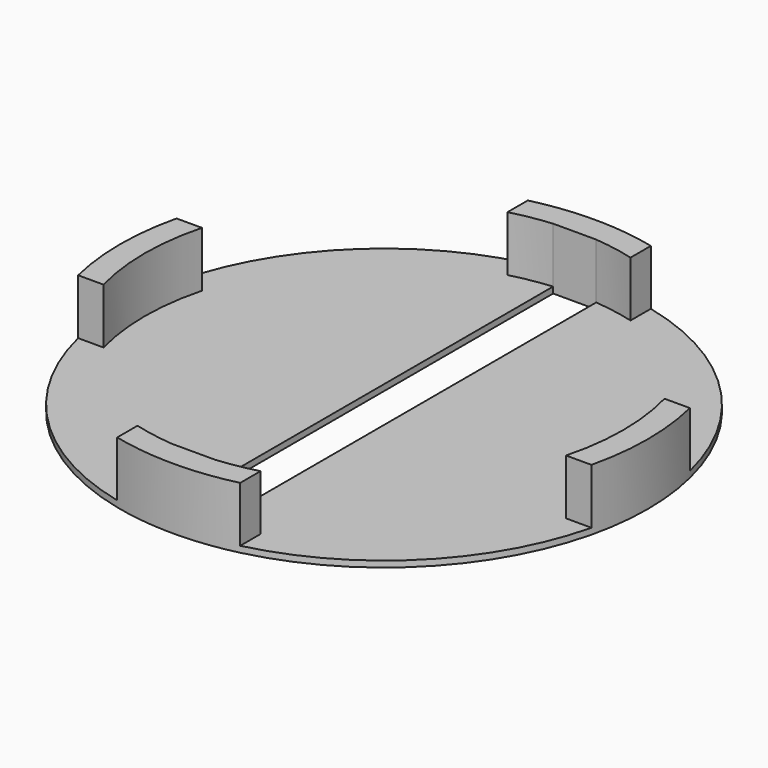
from build123d import *

# Parameters (mm, degrees)
F0_W     = 3.5
F0_H     = 1.4879982061
F0_W_2   = 3.25
F0_H_2   = 10
F0_H_3   = 0.5193831472
F1_DEPTH = 0.5
F2_DEPTH = 5


# Not quite as in the source:
# - a feature of the source that left no trace in its solid (it failed there, or was rolled back) is left out
# - a feature names something its author has since deleted; it is built from what else it names


with BuildPart() as f1:
    # F0 (on Top) → F1 (new body)
    with BuildSketch(Plane.XY):
        with BuildLine():
            Line((-1.75, 5), (-1.75, 19.3711125132))
            ThreePointArc((-1.75, 19.3711125132), (-3.3872134677, 19.1527879152), (-5, 18.7963427294))
            Line((-5, 18.7963427294), (-5, 5))
            Line((-5, 5), (-1.75, 5))
        make_face()
        with BuildLine():
            ThreePointArc((-5, 18.7963427294), (-3.3872134677, 19.1527879152), (-1.75, 19.3711125132))
            Line((-1.75, 19.3711125132), (-1.75, 20.8591107193))
            Line((-1.75, 20.8591107193), (-5, 20.8591107193))
            Line((-5, 20.8591107193), (-5, 18.7963427294))
        make_face()
        with Locations((0, 20.1151116163)):
            Rectangle(F0_W, F0_H)
        with BuildLine():
            Line((-5, 5), (-5, 18.7963427294))
            ThreePointArc((-5, 18.7963427294), (-13.7532268941, 13.7532268941), (-18.7963427294, 5))
            Line((-18.7963427294, 5), (-5, 5))
        make_face()
        with BuildLine():
            ThreePointArc((-18.7963427294, 5), (-13.7532268941, 13.7532268941), (-5, 18.7963427294))
            Line((-5, 18.7963427294), (-5, 20.8591107193))
            ThreePointArc((-5, 20.8591107193), (-15.1674404565, 15.1674404565), (-20.8591107193, 5))
            Line((-20.8591107193, 5), (-18.7963427294, 5))
        make_face()
        with Locations((-3.375, 0)):
            Rectangle(F0_W_2, F0_H_2)
        with Locations((0, 21.1188022929)):
            Rectangle(F0_W, F0_H_3)
        with BuildLine():
            Line((-5, 20.8591107193), (-1.75, 20.8591107193))
            Line((-1.75, 20.8591107193), (-1.75, 21.3784938665))
            ThreePointArc((-1.75, 21.3784938665), (-3.3849763239, 21.1812283706), (-5, 20.8591107193))
        make_face()
        with BuildLine():
            ThreePointArc((5, 18.7963427294), (3.3872134677, 19.1527879152), (1.75, 19.3711125132))
            Line((1.75, 19.3711125132), (1.75, 5))
            Line((1.75, 5), (5, 5))
            Line((5, 5), (5, 18.7963427294))
        make_face()
        with BuildLine():
            Line((1.75, 20.8591107193), (1.75, 19.3711125132))
            ThreePointArc((1.75, 19.3711125132), (3.3872134677, 19.1527879152), (5, 18.7963427294))
            Line((5, 18.7963427294), (5, 20.8591107193))
            Line((5, 20.8591107193), (1.75, 20.8591107193))
        make_face()
        with BuildLine():
            Line((-5, 5), (-18.7963427294, 5))
            ThreePointArc((-18.7963427294, 5), (-19.45, 0), (-18.7963427294, -5))
            Line((-18.7963427294, -5), (-5, -5))
            Line((-5, -5), (-5, 5))
        make_face()
        with BuildLine():
            ThreePointArc((-18.7963427294, -5), (-19.45, 0), (-18.7963427294, 5))
            Line((-18.7963427294, 5), (-20.8591107193, 5))
            Line((-20.8591107193, 5), (-20.8591107193, -5))
            Line((-20.8591107193, -5), (-18.7963427294, -5))
        make_face()
        with Locations((3.375, 0)):
            Rectangle(F0_W_2, F0_H_2)
        with BuildLine():
            Line((-1.75, -19.3711125132), (-1.75, -5))
            Line((-1.75, -5), (-5, -5))
            Line((-5, -5), (-5, -18.7963427294))
            ThreePointArc((-5, -18.7963427294), (-3.3872134677, -19.1527879152), (-1.75, -19.3711125132))
        make_face()
        with BuildLine():
            Line((1.75, 21.3784938665), (1.75, 20.8591107193))
            Line((1.75, 20.8591107193), (5, 20.8591107193))
            ThreePointArc((5, 20.8591107193), (3.3849763239, 21.1812283706), (1.75, 21.3784938665))
        make_face()
        with BuildLine():
            ThreePointArc((1.75, 21.3784938665), (0, 21.45), (-1.75, 21.3784938665))
            Line((-1.75, 21.3784938665), (1.75, 21.3784938665))
        make_face()
        with BuildLine():
            ThreePointArc((18.7963427294, 5), (13.7532268941, 13.7532268941), (5, 18.7963427294))
            Line((5, 18.7963427294), (5, 5))
            Line((5, 5), (18.7963427294, 5))
        make_face()
        with BuildLine():
            Line((5, 20.8591107193), (5, 18.7963427294))
            ThreePointArc((5, 18.7963427294), (13.7532268941, 13.7532268941), (18.7963427294, 5))
            Line((18.7963427294, 5), (20.8591107193, 5))
            ThreePointArc((20.8591107193, 5), (15.1674404565, 15.1674404565), (5, 20.8591107193))
        make_face()
        with BuildLine():
            Line((-5, -5), (-18.7963427294, -5))
            ThreePointArc((-18.7963427294, -5), (-13.7532268941, -13.7532268941), (-5, -18.7963427294))
            Line((-5, -18.7963427294), (-5, -5))
        make_face()
        with BuildLine():
            ThreePointArc((-5, -18.7963427294), (-13.7532268941, -13.7532268941), (-18.7963427294, -5))
            Line((-18.7963427294, -5), (-20.8591107193, -5))
            ThreePointArc((-20.8591107193, -5), (-15.1674404565, -15.1674404565), (-5, -20.8591107193))
            Line((-5, -20.8591107193), (-5, -18.7963427294))
        make_face()
        with BuildLine():
            Line((-20.8591107193, -5), (-20.8591107193, 5))
            ThreePointArc((-20.8591107193, 5), (-21.45, 0), (-20.8591107193, -5))
        make_face()
        with BuildLine():
            Line((18.7963427294, 5), (5, 5))
            Line((5, 5), (5, -5))
            Line((5, -5), (18.7963427294, -5))
            ThreePointArc((18.7963427294, -5), (19.45, 0), (18.7963427294, 5))
        make_face()
        with BuildLine():
            Line((5, -5), (1.75, -5))
            Line((1.75, -5), (1.75, -19.3711125132))
            ThreePointArc((1.75, -19.3711125132), (3.3872134677, -19.1527879152), (5, -18.7963427294))
            Line((5, -18.7963427294), (5, -5))
        make_face()
        with BuildLine():
            Line((-1.75, -20.8591107193), (-1.75, -19.3711125132))
            ThreePointArc((-1.75, -19.3711125132), (-3.3872134677, -19.1527879152), (-5, -18.7963427294))
            Line((-5, -18.7963427294), (-5, -20.8591107193))
            Line((-5, -20.8591107193), (-1.75, -20.8591107193))
        make_face()
        with Locations((0, -20.1151116163)):
            Rectangle(F0_W, F0_H)
        with BuildLine():
            Line((20.8591107193, 5), (18.7963427294, 5))
            ThreePointArc((18.7963427294, 5), (19.45, 0), (18.7963427294, -5))
            Line((18.7963427294, -5), (20.8591107193, -5))
            Line((20.8591107193, -5), (20.8591107193, 5))
        make_face()
        with BuildLine():
            Line((18.7963427294, -5), (5, -5))
            Line((5, -5), (5, -18.7963427294))
            ThreePointArc((5, -18.7963427294), (13.7532268941, -13.7532268941), (18.7963427294, -5))
        make_face()
        with BuildLine():
            ThreePointArc((5, -18.7963427294), (3.3872134677, -19.1527879152), (1.75, -19.3711125132))
            Line((1.75, -19.3711125132), (1.75, -20.8591107193))
            Line((1.75, -20.8591107193), (5, -20.8591107193))
            Line((5, -20.8591107193), (5, -18.7963427294))
        make_face()
        with BuildLine():
            Line((-1.75, -21.3784938665), (-1.75, -20.8591107193))
            Line((-1.75, -20.8591107193), (-5, -20.8591107193))
            ThreePointArc((-5, -20.8591107193), (-3.3849763239, -21.1812283706), (-1.75, -21.3784938665))
        make_face()
        with Locations((0, -21.1188022929)):
            Rectangle(F0_W, F0_H_3)
        with BuildLine():
            ThreePointArc((21.45, 0), (21.3017654776, 2.5173969761), (20.8591107193, 5))
            Line((20.8591107193, 5), (20.8591107193, -5))
            ThreePointArc((20.8591107193, -5), (21.3017654776, -2.5173969761), (21.45, 0))
        make_face()
        with BuildLine():
            Line((20.8591107193, -5), (18.7963427294, -5))
            ThreePointArc((18.7963427294, -5), (13.7532268941, -13.7532268941), (5, -18.7963427294))
            Line((5, -18.7963427294), (5, -20.8591107193))
            ThreePointArc((5, -20.8591107193), (15.1674404565, -15.1674404565), (20.8591107193, -5))
        make_face()
        with BuildLine():
            Line((5, -20.8591107193), (1.75, -20.8591107193))
            Line((1.75, -20.8591107193), (1.75, -21.3784938665))
            ThreePointArc((1.75, -21.3784938665), (3.3849763239, -21.1812283706), (5, -20.8591107193))
        make_face()
        with BuildLine():
            Line((1.75, -21.3784938665), (-1.75, -21.3784938665))
            ThreePointArc((-1.75, -21.3784938665), (0, -21.45), (1.75, -21.3784938665))
        make_face()
    extrude(amount=F1_DEPTH)

    # F0 (on Top) → F2 (join)
    with BuildSketch(Plane.XY):
        with BuildLine():
            ThreePointArc((-5, 18.7963427294), (-3.3872134677, 19.1527879152), (-1.75, 19.3711125132))
            Line((-1.75, 19.3711125132), (-1.75, 20.8591107193))
            Line((-1.75, 20.8591107193), (-5, 20.8591107193))
            Line((-5, 20.8591107193), (-5, 18.7963427294))
        make_face()
        with Locations((0, 20.1151116163)):
            Rectangle(F0_W, F0_H)
        with Locations((0, 21.1188022929)):
            Rectangle(F0_W, F0_H_3)
        with BuildLine():
            Line((-5, 20.8591107193), (-1.75, 20.8591107193))
            Line((-1.75, 20.8591107193), (-1.75, 21.3784938665))
            ThreePointArc((-1.75, 21.3784938665), (-3.3849763239, 21.1812283706), (-5, 20.8591107193))
        make_face()
        with BuildLine():
            Line((1.75, 20.8591107193), (1.75, 19.3711125132))
            ThreePointArc((1.75, 19.3711125132), (3.3872134677, 19.1527879152), (5, 18.7963427294))
            Line((5, 18.7963427294), (5, 20.8591107193))
            Line((5, 20.8591107193), (1.75, 20.8591107193))
        make_face()
        with BuildLine():
            ThreePointArc((-18.7963427294, -5), (-19.45, 0), (-18.7963427294, 5))
            Line((-18.7963427294, 5), (-20.8591107193, 5))
            Line((-20.8591107193, 5), (-20.8591107193, -5))
            Line((-20.8591107193, -5), (-18.7963427294, -5))
        make_face()
        with BuildLine():
            Line((1.75, 21.3784938665), (1.75, 20.8591107193))
            Line((1.75, 20.8591107193), (5, 20.8591107193))
            ThreePointArc((5, 20.8591107193), (3.3849763239, 21.1812283706), (1.75, 21.3784938665))
        make_face()
        with BuildLine():
            ThreePointArc((1.75, 21.3784938665), (0, 21.45), (-1.75, 21.3784938665))
            Line((-1.75, 21.3784938665), (1.75, 21.3784938665))
        make_face()
        with BuildLine():
            Line((-20.8591107193, -5), (-20.8591107193, 5))
            ThreePointArc((-20.8591107193, 5), (-21.45, 0), (-20.8591107193, -5))
        make_face()
        with BuildLine():
            Line((-1.75, -20.8591107193), (-1.75, -19.3711125132))
            ThreePointArc((-1.75, -19.3711125132), (-3.3872134677, -19.1527879152), (-5, -18.7963427294))
            Line((-5, -18.7963427294), (-5, -20.8591107193))
            Line((-5, -20.8591107193), (-1.75, -20.8591107193))
        make_face()
        with Locations((0, -20.1151116163)):
            Rectangle(F0_W, F0_H)
        with BuildLine():
            Line((20.8591107193, 5), (18.7963427294, 5))
            ThreePointArc((18.7963427294, 5), (19.45, 0), (18.7963427294, -5))
            Line((18.7963427294, -5), (20.8591107193, -5))
            Line((20.8591107193, -5), (20.8591107193, 5))
        make_face()
        with BuildLine():
            ThreePointArc((5, -18.7963427294), (3.3872134677, -19.1527879152), (1.75, -19.3711125132))
            Line((1.75, -19.3711125132), (1.75, -20.8591107193))
            Line((1.75, -20.8591107193), (5, -20.8591107193))
            Line((5, -20.8591107193), (5, -18.7963427294))
        make_face()
        with BuildLine():
            Line((-1.75, -21.3784938665), (-1.75, -20.8591107193))
            Line((-1.75, -20.8591107193), (-5, -20.8591107193))
            ThreePointArc((-5, -20.8591107193), (-3.3849763239, -21.1812283706), (-1.75, -21.3784938665))
        make_face()
        with Locations((0, -21.1188022929)):
            Rectangle(F0_W, F0_H_3)
        with BuildLine():
            ThreePointArc((21.45, 0), (21.3017654776, 2.5173969761), (20.8591107193, 5))
            Line((20.8591107193, 5), (20.8591107193, -5))
            ThreePointArc((20.8591107193, -5), (21.3017654776, -2.5173969761), (21.45, 0))
        make_face()
        with BuildLine():
            Line((5, -20.8591107193), (1.75, -20.8591107193))
            Line((1.75, -20.8591107193), (1.75, -21.3784938665))
            ThreePointArc((1.75, -21.3784938665), (3.3849763239, -21.1812283706), (5, -20.8591107193))
        make_face()
        with BuildLine():
            Line((1.75, -21.3784938665), (-1.75, -21.3784938665))
            ThreePointArc((-1.75, -21.3784938665), (0, -21.45), (1.75, -21.3784938665))
        make_face()
    extrude(amount=F2_DEPTH)


solid = f1.part
